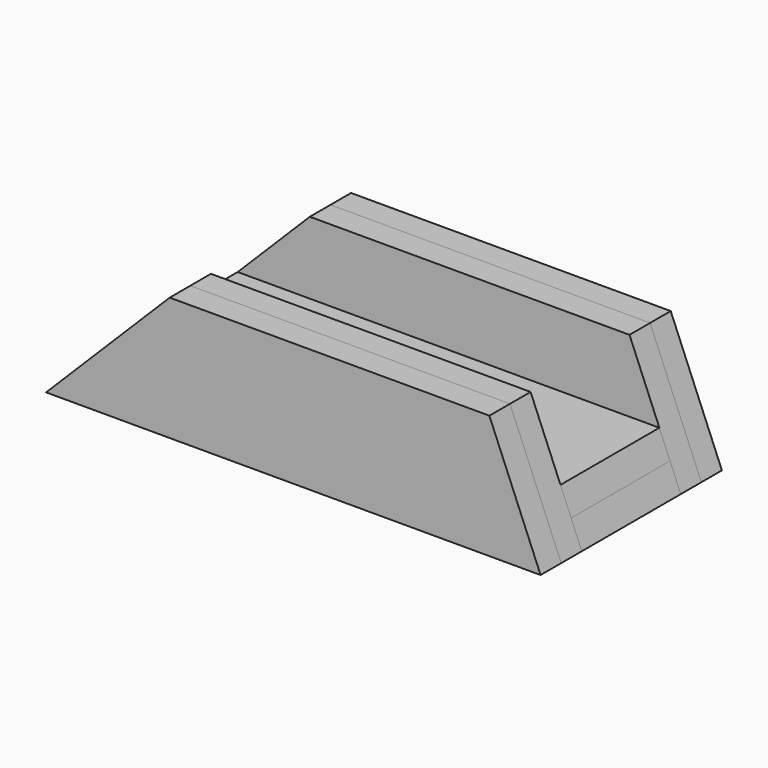
from build123d import *

# Parameters (mm, degrees)
F1_W          = 304.8
F1_H          = 76.2
F2_DEPTH      = 15.875
F5_W          = 304.8
F5_H          = 15.875
F6_DEPTH      = 76.2
F9_DEPTH      = 69.851
F9_DEPTH_BACK = 69.851


# Not quite as in the source:
# - a length typed as a fraction of an inch, garbled in the dataset ("3 / 203.2 mm" for 3/8 in), is restored


with BuildPart() as f2:
    # F1 (on offset) → F2 (new body)
    with BuildSketch(Plane.XZ.offset(38.1)):
        Rectangle(F1_W, F1_H)
    extrude(amount=F2_DEPTH)


with BuildPart() as f3_1:
    # F3: instance of F2
    add(f2.part.mirror(Plane.XZ.offset(53.975)))


with BuildPart() as f4_1:
    # F4: instance of F2
    add(f2.part.mirror(Plane.XZ))


with BuildPart() as f4_2:
    # F4: instance of F3_1
    add(f3_1.part.mirror(Plane.XZ))


with BuildPart() as f6:
    # F5 (on offset) → F6 (new body, through all)
    with BuildSketch(Plane.XZ.offset(38.1)):
        with Locations((0, -30.1625)):
            Rectangle(F5_W, F5_H)
    extrude(amount=-F6_DEPTH)


with BuildPart() as f7_1:
    # F7: instance of F6
    add(f6.part.mirror(Plane.XY.offset(-22.225)))


with BuildPart() as f9_tool:
    # F8 (on Front) → F9 (new body, two sides)
    with BuildSketch(Plane.XZ) as f9_sk:
        Polygon((-152.4, 38.1), (-152.4, -38.1), (-76.2, 38.1), align=None)
        Polygon((120.8369265472, 38.1), (152.4, -38.1), (152.4, 38.1), align=None)
    extrude(amount=-F9_DEPTH)
    extrude(f9_sk.sketch, amount=F9_DEPTH_BACK)


with BuildPart() as f2_1:
    add(f2.part)

    # F9: cut by f9_tool
    add(f9_tool.part, mode=Mode.SUBTRACT)


with BuildPart() as f3_1_1:
    add(f3_1.part)

    # F9: cut by f9_tool
    add(f9_tool.part, mode=Mode.SUBTRACT)


with BuildPart() as f4_1_1:
    add(f4_1.part)

    # F9: cut by f9_tool
    add(f9_tool.part, mode=Mode.SUBTRACT)


with BuildPart() as f4_2_1:
    add(f4_2.part)

    # F9: cut by f9_tool
    add(f9_tool.part, mode=Mode.SUBTRACT)


with BuildPart() as f6_1:
    add(f6.part)

    # F9: cut by f9_tool
    add(f9_tool.part, mode=Mode.SUBTRACT)


with BuildPart() as f7_1_1:
    add(f7_1.part)

    # F9: cut by f9_tool
    add(f9_tool.part, mode=Mode.SUBTRACT)


solid = Compound([f2_1.part, f3_1_1.part, f4_1_1.part, f4_2_1.part, f6_1.part, f7_1_1.part])
